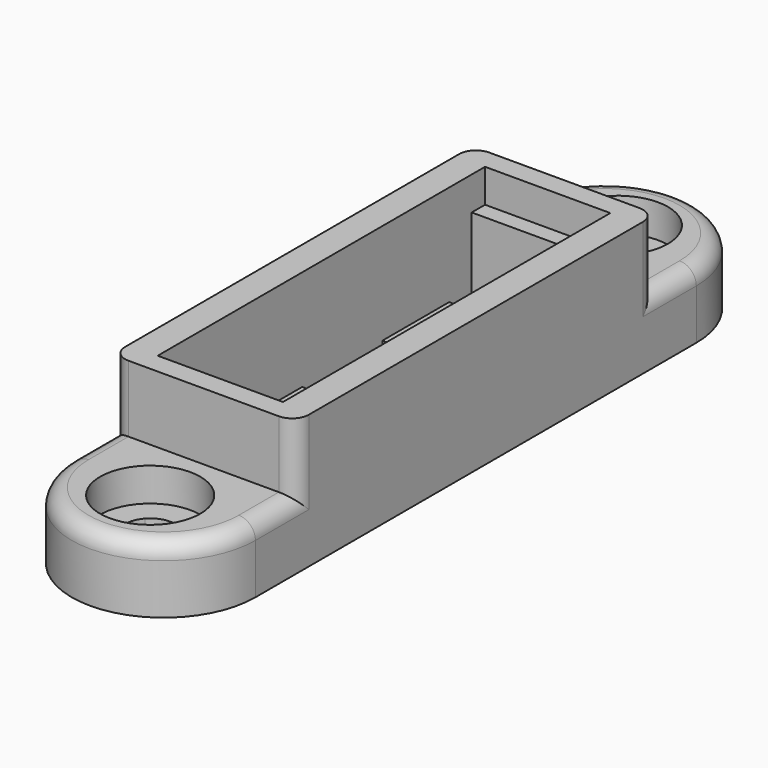
from build123d import *

# Parameters (mm, degrees)
F1_DEPTH  = 4
F2_W      = 11
F2_H      = 27
F3_DEPTH  = 4
F4_W      = 7.5
F4_H      = 24.5
F5_DEPTH  = 7
F6_W      = 7.5
F6_H      = 1
F7_DEPTH  = 5
F8_W      = 7.5
F8_H      = 2
F9_DEPTH  = 25
F10_W     = 5
F10_H     = 5
F11_DEPTH = 2
F12_R     = 3
F12_R_2   = 1.5
F13_DEPTH = 2
F14_R     = 1


# Not quite as in the source:
# - a feature names something its author has since deleted; it is built from what else it names


with BuildPart() as f1:
    # F0 (on Top) → F1 (new body)
    with BuildSketch(Plane.XY):
        with BuildLine():
            ThreePointArc((-5.5, -16.5), (0, -22), (5.5, -16.5))
            Line((5.5, -16.5), (1.1180339887, -16.5))
            ThreePointArc((1.1180339887, -16.5), (1.4012585384, -16.9647668653), (1.5, -17.5))
            ThreePointArc((1.5, -17.5), (-0.5352331347, -18.9012585384), (-1.1180339887, -16.5))
            Line((-1.1180339887, -16.5), (-5.5, -16.5))
        make_face()
        with BuildLine():
            Line((1.1180339887, -16.5), (5.5, -16.5))
            Line((5.5, -16.5), (5.5, 16.5))
            Line((5.5, 16.5), (1.1180339887, 16.5))
            ThreePointArc((1.1180339887, 16.5), (0, 16), (-1.1180339887, 16.5))
            Line((-1.1180339887, 16.5), (-5.5, 16.5))
            Line((-5.5, 16.5), (-5.5, -16.5))
            Line((-5.5, -16.5), (-1.1180339887, -16.5))
            ThreePointArc((-1.1180339887, -16.5), (0, -16), (1.1180339887, -16.5))
        make_face()
        with BuildLine():
            Line((1.1180339887, 16.5), (5.5, 16.5))
            ThreePointArc((5.5, 16.5), (0, 22), (-5.5, 16.5))
            Line((-5.5, 16.5), (-1.1180339887, 16.5))
            ThreePointArc((-1.1180339887, 16.5), (-0.5352331347, 18.9012585384), (1.5, 17.5))
            ThreePointArc((1.5, 17.5), (1.4012585384, 16.9647668653), (1.1180339887, 16.5))
        make_face()
    extrude(amount=F1_DEPTH)

    # F2 (on face) → F3 (join)
    with BuildSketch(Plane.XY.offset(4)):
        Rectangle(F2_W, F2_H)
    extrude(amount=F3_DEPTH)

    # F4 (on face) → F5 (cut)
    with BuildSketch(Plane.XY.offset(8)):
        Rectangle(F4_W, F4_H)
    extrude(amount=-F5_DEPTH, mode=Mode.SUBTRACT)

    # F6 (on face) → F7 (join)
    with BuildSketch(Plane.XY.offset(1)):
        with Locations((0, 11.75)):
            Rectangle(F6_W, F6_H)
        with Locations((0, -11.75)):
            Rectangle(F6_W, F6_H)
    extrude(amount=F7_DEPTH)

    # F8 (on face) → F9 (cut)
    with BuildSketch(Plane.XY.offset(1)):
        with Locations((0, 10.25)):
            Rectangle(F8_W, F8_H)
        with Locations((0, -10.25)):
            Rectangle(F8_W, F8_H)
    extrude(amount=-F9_DEPTH, mode=Mode.SUBTRACT)

    # F12 (on face) → F13 (cut)
    with BuildSketch(Plane.XY.offset(4)):
        with Locations((0, 17.5)):
            Circle(F12_R)
        with Locations((0, -17.5)):
            Circle(F12_R)
        with Locations((0, -17.5)):
            Circle(F12_R_2, mode=Mode.SUBTRACT)
    extrude(amount=-F13_DEPTH, mode=Mode.SUBTRACT)

    # F14
    f14_edges = [f1.edges().sort_by_distance(p)[0] for p in [
        (0, -22, 4),
        (-5.5, -13.5, 6),
        (5.5, -13.5, 6),
        (5.5, 13.5, 6),
        (-5.5, 13.5, 6),
        (0, 22, 4),
    ]]
    fillet(f14_edges, radius=F14_R)


with BuildPart() as f11:
    # F10 (on face) → F11 (new body)
    with BuildSketch(Plane.XY.offset(1)):
        with Locations((0, 5.5)):
            Rectangle(F10_W, F10_H)
    extrude(amount=F11_DEPTH)


with BuildPart() as f11b:
    # F10 (on face) → F11, piece 2 (new body)
    with BuildSketch(Plane.XY.offset(1)):
        with Locations((0, -5.5)):
            Rectangle(F10_W, F10_H)
    extrude(amount=F11_DEPTH)


solid = Compound([f1.part, f11.part, f11b.part])
